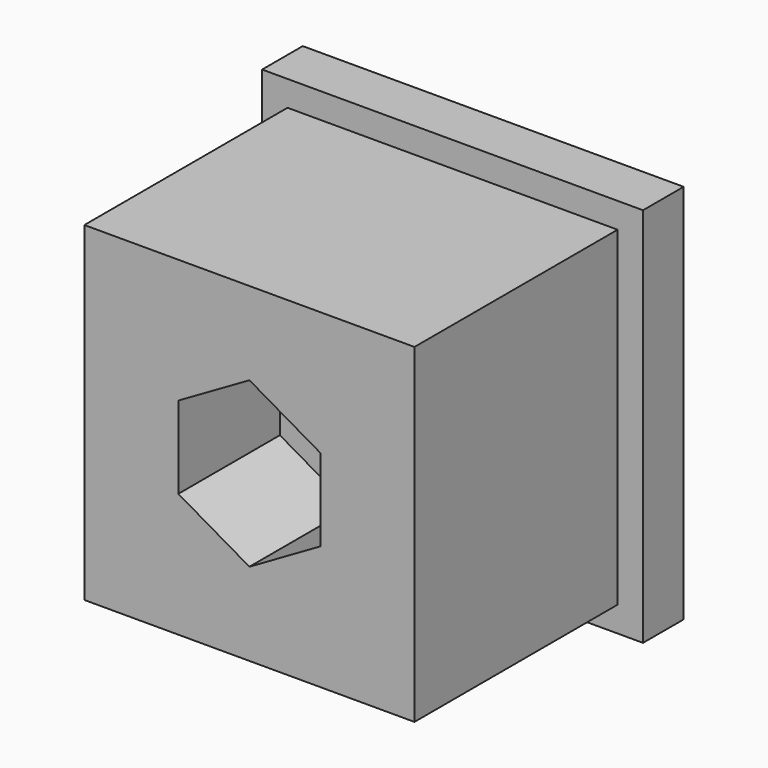
from build123d import *

# Parameters (mm, degrees)
F0_W     = 15
F0_H     = 15
F1_DEPTH = 2
F2_W     = 13
F2_H     = 13
F3_DEPTH = 10
F5_DEPTH = 12
F7_DEPTH = 5


# Not quite as in the source:
# - a feature names something its author has since deleted; it is built from what else it names


with BuildPart() as f1:
    # F0 (on Front) → F1 (new body)
    with BuildSketch(Plane.XZ):
        Rectangle(F0_W, F0_H)
    extrude(amount=F1_DEPTH)

    # F2 (on face) → F3 (join)
    with BuildSketch(Plane.XZ.offset(2)):
        Rectangle(F2_W, F2_H)
    extrude(amount=F3_DEPTH)

    # F4 (on face) → F5 (cut, through all)
    with BuildSketch(Plane(origin=(0, 0, 0), x_dir=(-1, 0, 0), z_dir=(0, 1, 0))):
        Polygon((1.5, -0.8660254038), (1.5, 0.8660254038), (0, 1.7320508076), (-1.5, 0.8660254038), (-1.5, -0.8660254038), (0, -1.7320508076), align=None)
    extrude(amount=-F5_DEPTH, mode=Mode.SUBTRACT)

    # F6 (on face) → F7 (cut)
    with BuildSketch(Plane.XZ.offset(12)):
        Polygon((-2.8, 1.6165807537), (-2.8, -1.6165807537), (0, -3.2331615075), (2.8, -1.6165807537), (2.8, 1.6165807537), (0, 3.2331615075), align=None)
        Polygon((1.5, 0.8660254038), (1.5, -0.8660254038), (0, -1.7320508076), (-1.5, -0.8660254038), (-1.5, 0.8660254038), (0, 1.7320508076), align=None, mode=Mode.SUBTRACT)
    extrude(amount=-F7_DEPTH, mode=Mode.SUBTRACT)


solid = f1.part
